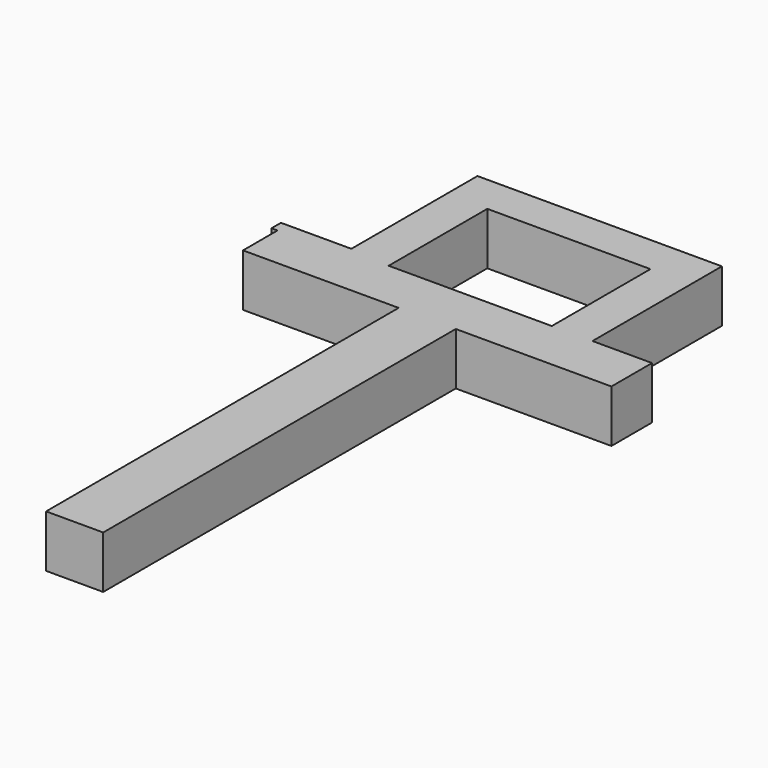
from build123d import *

# Parameters (mm, degrees)
F0_W     = 1.5524325391
F0_H     = 0.160164271
F0_W_2   = 2.4587620781
F0_H_2   = 0.2921586143
F0_W_3   = 2.2736147407
F0_W_4   = 3.1142332609
F0_W_5   = 2.4696406052
F0_W_6   = 0.6445926557
F1_DEPTH = 2


with BuildPart() as f1:
    # F0 (on Top) → F1 (new body)
    with BuildSketch(Plane.XY):
        Polygon((2.6887415443, 0), (0, 0), (0, -0.4523228854), (0.2299794661, -0.4523228854), (0.2299794661, -0.160164271), (2.6887415443, -0.160164271), align=None)
        Polygon((2.6887415443, 6.0171082268), (2.6887415443, 0), (4.2411740834, 0), (4.2411740834, 4.546245339), (7.3554073443, 4.546245339), (7.3554073443, 6.0171082268), align=None)
        with Locations((3.4649578138, -0.0800821355)):
            Rectangle(F0_W, F0_H)
        with Locations((1.4593605052, -0.3062435782)):
            Rectangle(F0_W_2, F0_H_2)
        Polygon((2.6887415443, -0.4523228854), (0.2299794661, -0.4523228854), (0.2299794661, -2.0985626283), (6.1724845996, -2.0985626283), (6.1724845996, -18.9240246407), (8.3531827515, -18.9240246407), (8.3531827515, -2.0985626283), (14.295687885, -2.0985626283), (14.295687885, -0.4523228854), (12.0220731443, -0.4523228854), (12.0220731443, -1.9231857732), (7.3554073443, -1.9231857732), (2.6887415443, -1.9231857732), align=None)
        Polygon((12.0220731443, 6.0171082268), (7.3554073443, 6.0171082268), (7.3554073443, 4.546245339), (10.4696406052, 4.546245339), (10.4696406052, 0), (12.0220731443, 0), align=None)
        with Locations((11.2458568747, -0.0800821355)):
            Rectangle(F0_W, F0_H)
        with Locations((11.2458568747, -0.3062435782)):
            Rectangle(F0_W, F0_H_2)
        with Locations((13.1588805146, -0.3062435782)):
            Rectangle(F0_W_3, F0_H_2)
        Polygon((8, -0.4523228854), (7.3554073443, -0.4523228854), (7.3554073443, -1.9231857732), (12.0220731443, -1.9231857732), (12.0220731443, -0.4523228854), (10.4696406052, -0.4523228854), align=None)
        Polygon((4.2411740834, -0.4523228854), (2.6887415443, -0.4523228854), (2.6887415443, -1.9231857732), (7.3554073443, -1.9231857732), (7.3554073443, -0.4523228854), align=None)
        with Locations((3.4649578138, -0.3062435782)):
            Rectangle(F0_W, F0_H_2)
        with Locations((5.7982907138, -0.3062435782)):
            Rectangle(F0_W_4, F0_H_2)
        with Locations((9.2348203026, -0.3062435782)):
            Rectangle(F0_W_5, F0_H_2)
        with Locations((7.6777036721, -0.3062435782)):
            Rectangle(F0_W_6, F0_H_2)
    extrude(amount=-F1_DEPTH)


solid = f1.part
